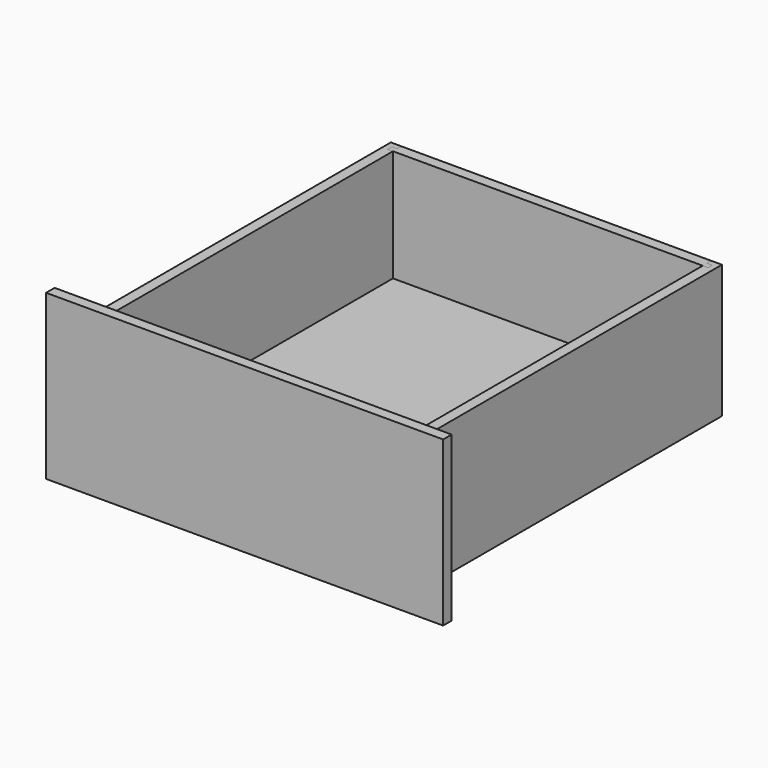
from build123d import *

# Parameters (mm, degrees)
F1_DEPTH  = 200
F2_DEPTH  = 200
F3_DEPTH  = 200
F4_DEPTH  = 200
F5_DEPTH  = 32
F7_DEPTH  = 561
F9_DEPTH  = 561
F10_W     = 596
F10_H     = 246
F10_W_2   = 465.0000002384
F10_H_2   = 200
F10_W_3   = 16
F10_W_4   = 15.9999997616
F11_DEPTH = 16


with BuildPart() as f1:
    # F0 (on Top) → F1 (new body)
    with BuildSketch(Plane.XY):
        Polygon((-248.5, -284.5), (-232.5000002384, -284.5), (-232.5000002384, -276.5000002384), (-240.5000002384, -276.5000002384), (-240.5000002384, -268.5000002384), (-232.5000002384, -268.5000002384), (-232.5000002384, 268.5000002384), (-240.5000002384, 268.5000002384), (-240.5000002384, 276.5000002384), (-232.5000002384, 276.5000002384), (-232.5000002384, 284.5), (-248.5, 284.5), align=None)
    extrude(amount=F1_DEPTH)


with BuildPart() as f2:
    # F0 (on Top) → F2 (new body)
    with BuildSketch(Plane.XY):
        Polygon((232.5, -284.5), (248.5, -284.5), (248.5, 284.5), (232.5, 284.5), (232.5, 276.5000002384), (240.5, 276.5000002384), (240.5, 268.5000002384), (232.5, 268.5000002384), (232.5, -268.5000002384), (240.5, -268.5000002384), (240.5, -276.5000002384), (232.5, -276.5000002384), align=None)
    extrude(amount=F2_DEPTH)


with BuildPart() as f3:
    # F0 (on Top) → F3 (new body)
    with BuildSketch(Plane.XY):
        Polygon((232.5, 276.5000002384), (232.5, 284.5), (-232.5000002384, 284.5), (-232.5000002384, 276.5000002384), (-240.5000002384, 276.5000002384), (-240.5000002384, 268.5000002384), (-232.5000002384, 268.5000002384), (232.5, 268.5000002384), (240.5, 268.5000002384), (240.5, 276.5000002384), align=None)
    extrude(amount=F3_DEPTH)

    # F0 (on Top) → F5 (cut)
    with BuildSketch(Plane.XY):
        Polygon((232.5, 276.5000002384), (232.5, 284.5), (-232.5000002384, 284.5), (-232.5000002384, 276.5000002384), (-240.5000002384, 276.5000002384), (-240.5000002384, 268.5000002384), (-232.5000002384, 268.5000002384), (232.5, 268.5000002384), (240.5, 268.5000002384), (240.5, 276.5000002384), align=None)
    extrude(amount=F5_DEPTH, mode=Mode.SUBTRACT)


with BuildPart() as f4:
    # F0 (on Top) → F4 (new body)
    with BuildSketch(Plane.XY):
        Polygon((-232.5000002384, -284.5), (232.5, -284.5), (232.5, -276.5000002384), (240.5, -276.5000002384), (240.5, -268.5000002384), (232.5, -268.5000002384), (-232.5000002384, -268.5000002384), (-240.5000002384, -268.5000002384), (-240.5000002384, -276.5000002384), (-232.5000002384, -276.5000002384), align=None)
    extrude(amount=F4_DEPTH)


with BuildPart() as f7:
    # F6 (on face) → F7 (new body)
    with BuildSketch(Plane(origin=(0, 284.5, 0), x_dir=(-1, 0, 0), z_dir=(0, 1, 0))):
        Polygon((-232.5, 32), (-240.5, 32), (-240.5, 16), (240.5000002384, 16), (240.5000002384, 32), (232.5000002384, 32), align=None)
    extrude(amount=-F7_DEPTH)


with BuildPart() as f2_1:
    add(f2.part)

    # F8: cut F7
    add(f7.part, mode=Mode.SUBTRACT)


with BuildPart() as f1_1:
    add(f1.part)

    # F8: cut F7
    add(f7.part, mode=Mode.SUBTRACT)


with BuildPart() as f4_1:
    add(f4.part)

    # F8: cut F7
    add(f7.part, mode=Mode.SUBTRACT)


with BuildPart() as f9:
    # F6 (on face) → F9 (new body)
    with BuildSketch(Plane(origin=(0, 284.5, 0), x_dir=(-1, 0, 0), z_dir=(0, 1, 0))):
        Polygon((-232.5, 32), (-240.5, 32), (-240.5, 16), (240.5000002384, 16), (240.5000002384, 32), (232.5000002384, 32), align=None)
    extrude(amount=-F9_DEPTH)


with BuildPart() as f11:
    # F10 (on face) → F11 (new body)
    with BuildSketch(Plane.XZ.offset(284.5)):
        with Locations((0, 100)):
            Rectangle(F10_W, F10_H)
        Polygon((-248.5, 0), (-248.5, 200), (-232.5000002384, 200), (232.5, 200), (248.5, 200), (248.5, 0), (232.5, 0), (-232.5000002384, 0), align=None, mode=Mode.SUBTRACT)
        with Locations((-1.192e-07, 100)):
            Rectangle(F10_W_2, F10_H_2)
        with Locations((240.5, 100)):
            Rectangle(F10_W_3, F10_H_2)
        with Locations((-240.5000001192, 100)):
            Rectangle(F10_W_4, F10_H_2)
    extrude(amount=F11_DEPTH)


solid = Compound([f3.part, f2_1.part, f1_1.part, f4_1.part, f9.part, f11.part])
